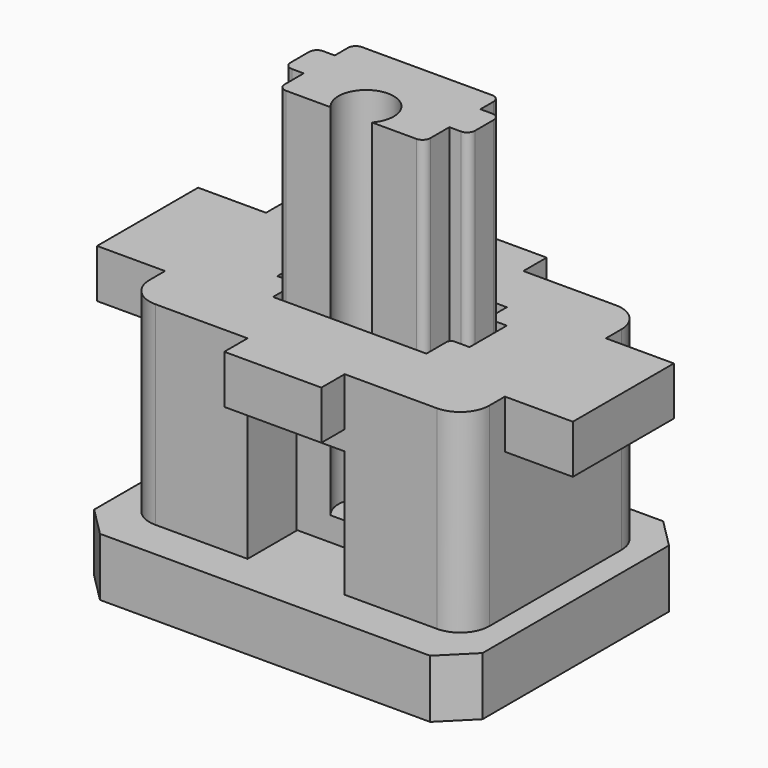
from build123d import *

# Parameters (mm, degrees)
F1_DEPTH  = 39
F2_W      = 40
F2_H      = 30
F3_DEPTH  = 6
F4_W      = 2
F4_H      = 4
F5_DEPTH  = 39
F6_R      = 0.8
F7_W      = 35
F7_H      = 23
F8_DEPTH  = 20
F9_R      = 3
F10_W     = 10
F10_H     = 3
F11_DEPTH = 5
F12_SIZE  = 3
F13_W     = 30
F13_H     = 0.6
F14_DEPTH = 10
F15_W     = 10
F15_H     = 15
F16_DEPTH = 13
F17_W     = 30
F17_H     = 0.7
F18_DEPTH = 1
F19_DEPTH = 2
F20_R     = 1.5
F21_DEPTH = 25
F22_W     = 7
F22_H     = 13
F23_DEPTH = 5
F24_SIZE  = 0.3


with BuildPart() as f1:
    # F0 (on Top) → F1 (new body)
    with BuildSketch(Plane.XY):
        with BuildLine():
            Line((7.5, 7.85), (-7.5, 7.85))
            Line((-7.5, 7.85), (-7.5, -1.9))
            Line((-7.5, -1.9), (-2.1242645786, -1.9))
            ThreePointArc((-2.1242645786, -1.9), (0, 2.85), (2.1242645786, -1.9))
            Line((2.1242645786, -1.9), (7.5, -1.9))
            Line((7.5, -1.9), (7.5, 7.85))
        make_face()
    extrude(amount=F1_DEPTH)

    # F2 (on face) → F3 (join)
    with BuildSketch(Plane(origin=(0, 0, 0), x_dir=(1, 0, 0), z_dir=(0, 0, -1))):
        with Locations((0, -2)):
            Rectangle(F2_W, F2_H)
    extrude(amount=F3_DEPTH)

    # F4 (on face) → F5 (join, through all)
    with BuildSketch(Plane.XY):
        with Locations((-8.5, 3.35)):
            Rectangle(F4_W, F4_H)
        with Locations((8.5, 3.35)):
            Rectangle(F4_W, F4_H)
    extrude(amount=F5_DEPTH)

    # F6
    f6_edges = [f1.edges().sort_by_distance(p)[0] for p in [
        (-7.5, -1.9, 19.5),
        (7.5, -1.9, 19.5),
        (7.5, 7.85, 19.5),
        (-7.5, 7.85, 19.5),
        (-9.5, 5.35, 19.5),
        (-9.5, 1.35, 19.5),
        (9.5, 1.35, 19.5),
        (9.5, 5.35, 19.5),
    ]]
    fillet(f6_edges, radius=F6_R)

    # F12
    f12_edges = [f1.edges().sort_by_distance(p)[0] for p in [
        (-20, -13, -3),
        (20, -13, -3),
        (20, 17, -3),
        (-20, 17, -3),
    ]]
    chamfer(f12_edges, length=F12_SIZE)

    # F17 (on face) → F18 (cut)
    with BuildSketch(Plane.XY):
        with Locations((0, -2.25)):
            Rectangle(F17_W, F17_H)
    extrude(amount=-F18_DEPTH, mode=Mode.SUBTRACT)

    # F19 (add): a face of the model
    f19_faces = [f1.faces().sort_by_distance(p)[0] for p in [
        (0, 0.2812457246, 0),
    ]]
    extrude(f19_faces, amount=F19_DEPTH)

    # F20 (on face) → F21 (cut)
    with BuildSketch(Plane.XY.offset(2)):
        Circle(F20_R)
    extrude(amount=-F21_DEPTH, mode=Mode.SUBTRACT)


with BuildPart() as f8:
    # F7 (on face) → F8 (new body)
    with BuildSketch(Plane.XY):
        with Locations((0, 2.5)):
            Rectangle(F7_W, F7_H)
        Polygon((-7.9, 5.75), (-7.9, 8.25), (7.9, 8.25), (7.9, 5.75), (9.9, 5.75), (9.9, 0.95), (7.9, 0.95), (7.9, -2.1), (-7.9, -2.1), (-7.9, 0.95), (-9.9, 0.95), (-9.9, 5.75), align=None, mode=Mode.SUBTRACT)
    extrude(amount=F8_DEPTH)

    # F9
    f9_edges = [f8.edges().sort_by_distance(p)[0] for p in [
        (17.5, 14, 10),
        (-17.5, 14, 10),
        (-17.5, -9, 10),
        (17.5, -9, 10),
    ]]
    fillet(f9_edges, radius=F9_R)

    # F10 (on face) → F11 (join)
    with BuildSketch(Plane.XY.offset(20)):
        with Locations((0, 15.5)):
            Rectangle(F10_W, F10_H)
        with Locations((0, -10.5)):
            Rectangle(F10_W, F10_H)
    extrude(amount=-F11_DEPTH)

    # F13 (on face) → F14 (cut)
    with BuildSketch(Plane(origin=(0, 0, 0), x_dir=(1, 0, 0), z_dir=(0, 0, -1))):
        with Locations((0, 2.4)):
            Rectangle(F13_W, F13_H)
    extrude(amount=-F14_DEPTH, mode=Mode.SUBTRACT)

    # F15 (on face) → F16 (cut)
    with BuildSketch(Plane(origin=(0, 0, 0), x_dir=(1, 0, 0), z_dir=(0, 0, -1))):
        with Locations((0, 7.5)):
            Rectangle(F15_W, F15_H)
    extrude(amount=-F16_DEPTH, mode=Mode.SUBTRACT)

    # F22 (on face) → F23 (join)
    with BuildSketch(Plane.XY.offset(20)):
        with Locations((-21, 2.5)):
            Rectangle(F22_W, F22_H)
        with Locations((21, 2.5)):
            Rectangle(F22_W, F22_H)
    extrude(amount=-F23_DEPTH)

    # F24
    f24_edges = [f8.edges().sort_by_distance(p)[0] for p in [
        (-7.9, 5.75, 10),
        (7.9, 5.75, 10),
        (-7.9, 0.95, 10),
        (7.9, 0.95, 10),
    ]]
    chamfer(f24_edges, length=F24_SIZE)


solid = Compound([f1.part, f8.part])
